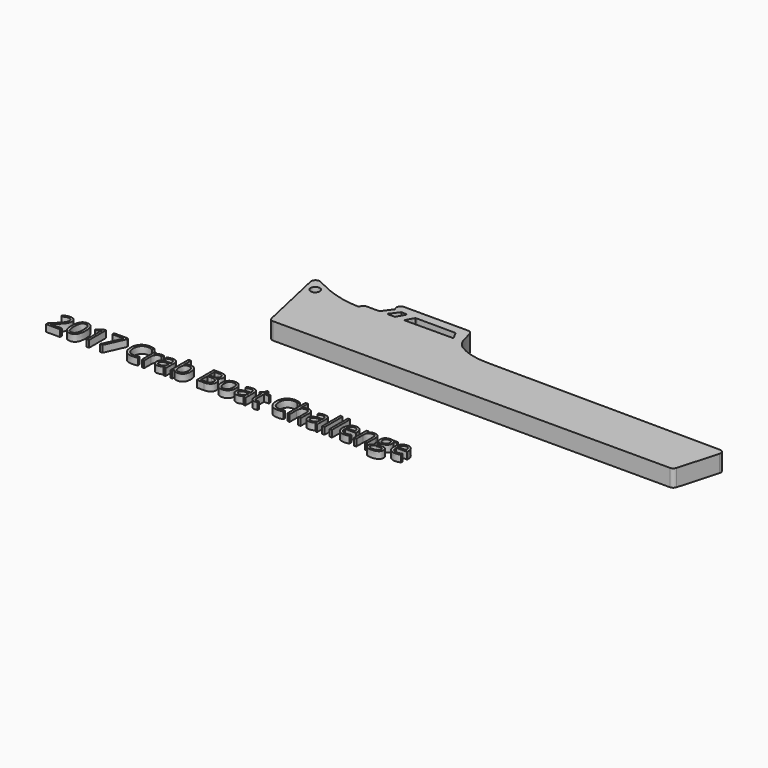
from build123d import *

# Parameters (mm, degrees)
F0_R         = 1.7144531012
F2_DEPTH     = 6.35
F1_TEXT_SIZE = 11.0718474995
F3_DEPTH     = 2.54


# Not quite as in the source:
# - Text() gives the source's letters only with a copy of the font that has no kerning and outlines rounded to 1/6400 em; it was checked with that copy


with BuildPart() as f2:
    # F0 (on Top) → F2 (new body)
    with BuildSketch(Plane.XY):
        with BuildLine():
            ThreePointArc((-82.6578963548, 16.6351178779), (-84.3524050739, 16.4782032173), (-84.9313041555, 14.8779351576))
            Line((-84.9313041555, 14.8779351576), (-79.3758570051, -10.1331158304))
            ThreePointArc((-79.3758570051, -10.1331158304), (-78.8195291366, -11.0271579858), (-77.826126409, -11.3763901348))
            Line((-77.826126409, -11.3763901348), (69.7269539483, -11.3763901348))
            ThreePointArc((69.7269539483, -11.3763901348), (70.6839738092, -11.0554876382), (71.254083355, -10.2225167311))
            Line((71.254083355, -10.2225167311), (75.4562824837, 4.5766259358))
            ThreePointArc((75.4562824837, 4.5766259358), (75.19873204, 5.9633136564), (73.9390647666, 6.5977215896))
            Line((73.9390647666, 6.5977215896), (-11.3526463776, 7.130257934))
            add(Edge.make_bspline(
                [(-12.8668220646, 7.1397120014), (-12.372094858, 7.1289012328), (-11.8671693523, 7.1257865528), (-11.3526463776, 7.130257934)],
                knots=[0.4231373007, 0.4231373007, 0.4231373007, 0.4231373007, 0.4697559219, 0.4697559219, 0.4697559219, 0.4697559219], degree=3))
            add(Edge.make_bspline(
                [(-24.3954672646, 10.0651517198), (-21.0074985022, 7.9699973196), (-17.3572494873, 7.2378367273), (-12.8668220646, 7.1397120014)],
                knots=[0, 0, 0, 0, 0.4231373007, 0.4231373007, 0.4231373007, 0.4231373007], degree=3))
            add(Edge.make_bspline(
                [(-28.386289363, 18.2088658517), (-27.5680035145, 14.8439996122), (-27.0323755451, 11.694124655), (-24.3954672646, 10.0651517198)],
                knots=[0.0520925717, 0.0520925717, 0.0520925717, 0.0520925717, 0.4883396262, 0.4883396262, 0.4883396262, 0.4883396262], degree=3))
            ThreePointArc((-28.386289363, 18.2088658517), (-28.9478512317, 19.0818737964), (-29.9288322239, 19.4212421755))
            Line((-29.9288322239, 19.4212421755), (-46.1653646044, 19.4212421755))
            add(Edge.make_bspline(
                [(-46.1891002262, 16.0552153603), (-45.8007262833, 16.4726439919), (-45.170890508, 17.5631013885), (-45.5943751344, 18.7109734238), (-46.1653646044, 19.4212421755)],
                knots=[0.6051427411, 0.6051427411, 0.6051427411, 0.6051427411, 0.646637232, 0.7098733844, 0.7098733844, 0.7098733844, 0.7098733844], degree=3))
            Line((-46.1891002262, 16.0552153603), (-31.8741314113, 15.990441665))
            Line((-31.8741314113, 15.990441665), (-30.251037274, 13.0147728891))
            Line((-30.251037274, 13.0147728891), (-48.5709768547, 12.9124532739))
            Line((-48.5709768547, 12.9124532739), (-47.355101634, 15.0968942509))
            add(Edge.make_bspline(
                [(-51.8151050758, 13.1146471412), (-50.0243845057, 13.6812317066), (-48.4772240612, 14.3547573158), (-47.355101634, 15.0968942509)],
                knots=[0.493608635, 0.493608635, 0.493608635, 0.493608635, 0.5723926752, 0.5723926752, 0.5723926752, 0.5723926752], degree=3))
            Line((-51.8151050758, 13.1146471412), (-51.9381151423, 12.8936473007))
            Line((-51.9381151423, 12.8936473007), (-52.5564191218, 12.89019398))
            add(Edge.make_bspline(
                [(-64.1152808122, 11.3057810813), (-60.2915866445, 11.268947734), (-56.0377535586, 11.8817545575), (-52.5564191218, 12.89019398)],
                knots=[0.3349455176, 0.3349455176, 0.3349455176, 0.3349455176, 0.4829274162, 0.4829274162, 0.4829274162, 0.4829274162], degree=3))
            add(Edge.make_bspline(
                [(-82.6578963548, 16.6351178779), (-77.1639177835, 13.8212551878), (-71.4257434064, 11.3762021967), (-64.1152808122, 11.3057810813)],
                knots=[0.0520211814, 0.0520211814, 0.0520211814, 0.0520211814, 0.3349455176, 0.3349455176, 0.3349455176, 0.3349455176], degree=3))
        make_face()
        with Locations((-80.698594451, 11.7666525766)):
            Circle(F0_R, mode=Mode.SUBTRACT)
        with BuildLine():
            Line((-63.9558078515, 11.7798734638), (-64.1152808122, 11.3057810813))
            add(Edge.make_bspline(
                [(-64.1152808122, 11.3057810813), (-60.2915866445, 11.268947734), (-56.0377535586, 11.8817545575), (-52.5564191218, 12.89019398)],
                knots=[0.3349455176, 0.3349455176, 0.3349455176, 0.3349455176, 0.4829274162, 0.4829274162, 0.4829274162, 0.4829274162], degree=3))
            Line((-52.5564191218, 12.89019398), (-54.9355708063, 12.8769060604))
            Line((-54.9355708063, 12.8769060604), (-52.3232373834, 16.3812569725))
            Line((-52.3232373834, 16.3812569725), (-50.0494301007, 16.2868581559))
            Line((-50.0494301007, 16.2868581559), (-51.8151050758, 13.1146471412))
            add(Edge.make_bspline(
                [(-51.8151050758, 13.1146471412), (-50.0243845057, 13.6812317066), (-48.4772240612, 14.3547573158), (-47.355101634, 15.0968942509)],
                knots=[0.493608635, 0.493608635, 0.493608635, 0.493608635, 0.5723926752, 0.5723926752, 0.5723926752, 0.5723926752], degree=3))
            Line((-47.355101634, 15.0968942509), (-46.8201041222, 16.0580705851))
            Line((-46.8201041222, 16.0580705851), (-46.1891002262, 16.0552153603))
            add(Edge.make_bspline(
                [(-46.1891002262, 16.0552153603), (-45.8007262833, 16.4726439919), (-45.170890508, 17.5631013885), (-45.5943751344, 18.7109734238), (-46.1653646044, 19.4212421755)],
                knots=[0.6051427411, 0.6051427411, 0.6051427411, 0.6051427411, 0.646637232, 0.7098733844, 0.7098733844, 0.7098733844, 0.7098733844], degree=3))
            Line((-46.1653646044, 19.4212421755), (-53.7738942729, 19.4212421755))
            ThreePointArc((-53.7738942729, 19.4212421755), (-55.116215914, 18.6812850133), (-55.2071857286, 17.1512234189))
            Line((-55.2071857286, 17.1512234189), (-54.9355708063, 16.5808312595))
            Line((-54.9355708063, 16.5808312595), (-57.7083528042, 12.8612443805))
            Line((-57.7083528042, 12.8612443805), (-62.4511518772, 12.8612443805))
            ThreePointArc((-62.4511518772, 12.8612443805), (-63.3776172922, 12.5628596138), (-63.9558078515, 11.7798734638))
        make_face()
    extrude(amount=F2_DEPTH)


with BuildPart() as f3:
    # F1 (on Top) → F3 (new body)
    with BuildSketch(Plane.XY):
        with Locations((-133.2894741087, -48.2921612129)):
            Text('2017 Crab Boat Challenge', F1_TEXT_SIZE, font='Open Sans', text_align=(TextAlign.LEFT, TextAlign.BOTTOM))
    extrude(amount=F3_DEPTH)


solid = Compound([f2.part, f3.part])
